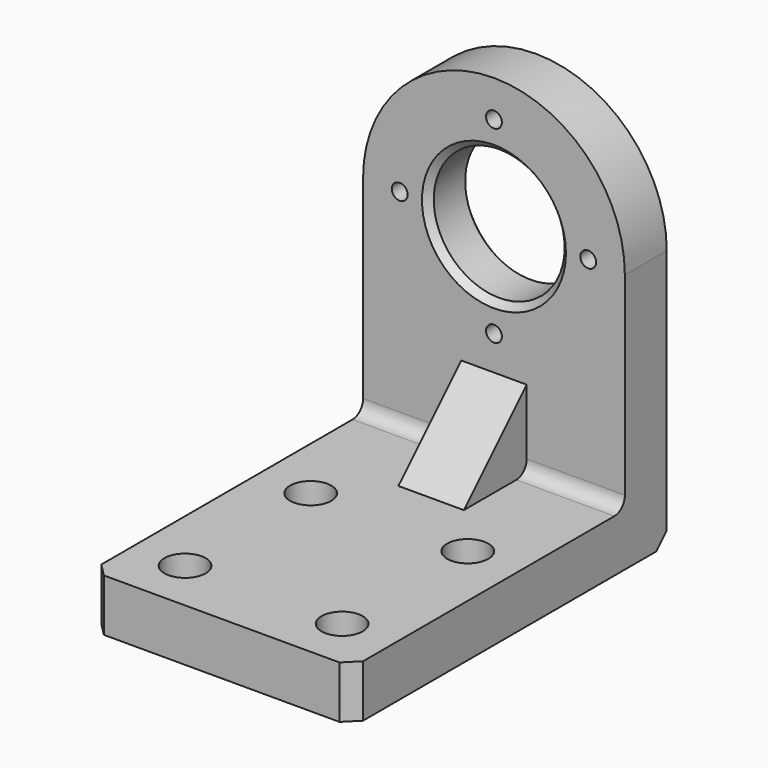
from build123d import *

# Parameters (mm, degrees)
F0_R           = 50
F1_DEPTH       = 40
F2_D           = 12.1
F3_W           = 50
F3_H           = 100
F4_DEPTH       = 40
F5_D           = 17.5
F5_CBORE_D     = 31.5
F5_CBORE_DEPTH = 20
F7_DEPTH       = 25
F8_SIZE        = 5
F9_SIZE        = 10
F10_R          = 10


# Not quite as in the source:
# - a feature names something its author has since deleted; it is built from what else it names


with BuildPart() as f1:
    # F0 (on Front) → F1 (new body)
    with BuildSketch(Plane.XZ):
        with BuildLine():
            Line((-100, 158.1762170792), (-100, 0))
            Line((-100, 0), (100, 0))
            Line((100, 0), (100, 158.1762170792))
            ThreePointArc((100, 158.1762170792), (0, 58.1762170792), (-100, 158.1762170792))
        make_face()
        Polygon((-100, -40), (0, -40), (100, -40), (100, 0), (-100, 0), align=None)
        with BuildLine():
            ThreePointArc((100, 158.1762170792), (0, 258.1762170792), (-100, 158.1762170792))
            ThreePointArc((-100, 158.1762170792), (0, 58.1762170792), (100, 158.1762170792))
        make_face()
        with Locations((0, 158.1762170792)):
            Circle(F0_R, mode=Mode.SUBTRACT)
    extrude(amount=-F1_DEPTH)

    # F2 (through all)
    with Locations(Plane.XZ):
        with Locations((-72, 158.1762170792), (0, 230.1762170792), (71.9880287234, 159.4891224521), (0, 86.1762170792)):
            Hole(F2_D / 2)

    # F3 (on Top) → F4 (join)
    with BuildSketch(Plane.XY):
        Polygon((-25, 40), (-100, 40), (-100, -220), (-100, -260), (100, -260), (100, -220), (100, 40), (25, 40), (25, -60), (-25, -60), align=None)
        with Locations((0, -10)):
            Rectangle(F3_W, F3_H)
    extrude(amount=-F4_DEPTH)

    # F5 (through all)
    with Locations(Plane.XY):
        with Locations((-60, -100), (60, -100), (60, -220), (-60, -220)):
            CounterBoreHole(F5_D / 2, F5_CBORE_D / 2, F5_CBORE_DEPTH)

    # F6 (on Right) → F7 (join, symmetric)
    with BuildSketch(Plane.YZ):
        Polygon((-60, 0), (0, 0), (0, 60), align=None)
    extrude(amount=F7_DEPTH, both=True)

    # F8
    f8_edges = [f1.edges().sort_by_distance(p)[0] for p in [
        (-50, 0, 158.176217),
        (-50, 40, 158.176217),
    ]]
    chamfer(f8_edges, length=F8_SIZE)

    # F9
    f9_edges = [f1.edges().sort_by_distance(p)[0] for p in [
        (0, 40, -40),
        (-100, -260, -20),
        (100, -260, -20),
    ]]
    chamfer(f9_edges, length=F9_SIZE)

    # F10
    f10_edges = [f1.edges().sort_by_distance(p)[0] for p in [
        (-62.5, 0, 0),
        (62.5, 0, 0),
    ]]
    fillet(f10_edges, radius=F10_R)


solid = f1.part
